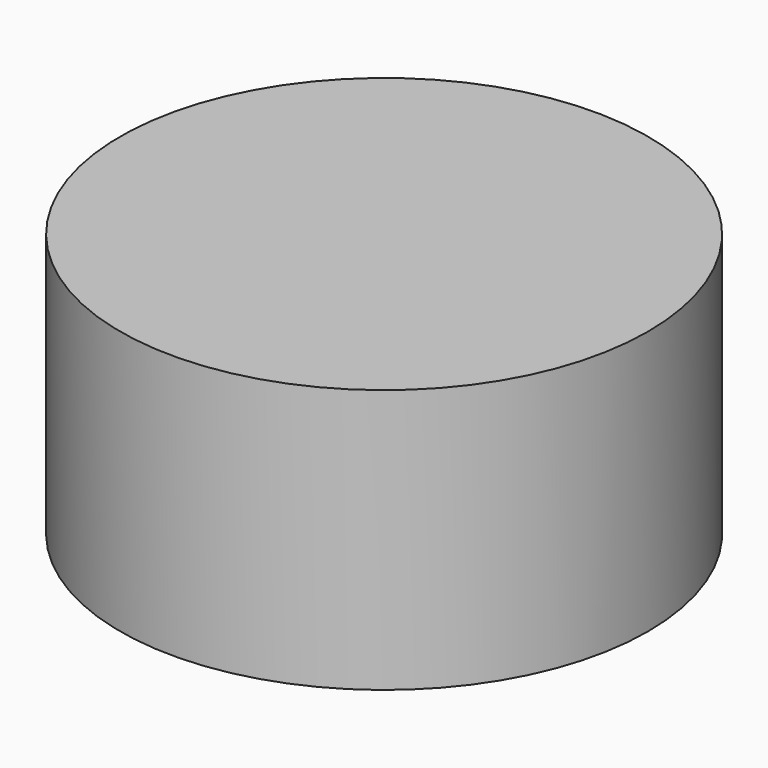
from build123d import *

# Parameters (mm, degrees)
F0_R     = 3.175
F3_DEPTH = 3.175


# Not quite as in the source:
# - the program builds the solid bodies; features that only make, move or delete a surface that nothing else refers to are left out


with BuildPart() as f3:
    # F0 (on Top) → F3 (new body)
    with BuildSketch(Plane.XY):
        Circle(F0_R)
    extrude(amount=F3_DEPTH)


solid = f3.part
